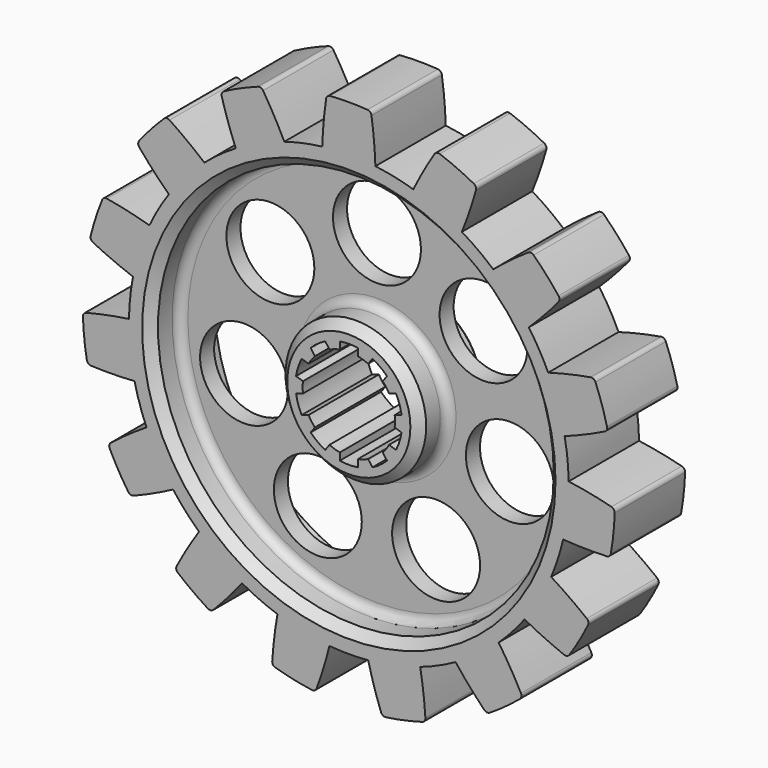
from build123d import *

# Parameters (mm, degrees)
F1_DEPTH  = 20
F2_DEPTH  = 20
F3_R      = 1
F4_COUNT  = 15
F5_R      = 10
F6_DEPTH  = 25
F7_R      = 45
F7_R_2    = 10
F7_R_3    = 16
F8_DEPTH  = 8
F9_R      = 2
F10_SIZE  = 2
F11_R     = 45
F11_R_2   = 16
F12_DEPTH = 8
F13_SIZE  = 2
F14_R     = 2


with BuildPart() as f1:
    # F0 (on Front) → F1 (new body)
    with BuildSketch(Plane.XZ):
        with BuildLine():
            ThreePointArc((-6.0454455831, 49.6331803102), (0, 50), (6.0454455831, 49.6331803102))
            ThreePointArc((6.0454455831, 49.6331803102), (5.6999328162, 54.9765582241), (5.0372687356, 60.2899321917))
            ThreePointArc((5.0372687356, 60.2899321917), (0, 60.5), (-5.0372687356, 60.2899321917))
            ThreePointArc((-5.0372687356, 60.2899321917), (-5.6999328162, 54.9765582241), (-6.0454455831, 49.6331803102))
        make_face()
    extrude(amount=F1_DEPTH)

    # F3
    f3_edges = [f1.edges().sort_by_distance(p)[0] for p in [
        (-5.037269, -10, 60.289932),
        (5.037269, -10, 60.289932),
    ]]
    fillet(f3_edges, radius=F3_R)



with BuildPart() as f2:
    # F0 (on Front) → F2 (new body)
    with BuildSketch(Plane.XZ):
        with BuildLine():
            ThreePointArc((-6.0454455831, 49.6331803102), (-33.14911553, -37.4317530925), (50, 0))
            ThreePointArc((50, 0), (37.4317530925, 33.14911553), (6.0454455831, 49.6331803102))
            ThreePointArc((6.0454455831, 49.6331803102), (0, 50), (-6.0454455831, 49.6331803102))
        make_face()
        with BuildLine():
            ThreePointArc((10.4274046286, 1.2325715847), (10.4818354452, 0.6173537882), (10.5, 0))
            ThreePointArc((10.5, 0), (10.4818354452, -0.6173537882), (10.4274046286, -1.2325715847))
            Line((10.4274046286, -1.2325715847), (11.9961998639, -1.742304056))
            ThreePointArc((11.9961998639, -1.742304056), (11.5230272808, -3.7440585238), (10.729230187, -5.6416357729))
            Line((10.729230187, -5.6416357729), (9.1604349517, -5.1319033015))
            ThreePointArc((9.1604349517, -5.1319033015), (8.4946784409, -6.1717451491), (7.7114601519, -7.1262460192))
            Line((7.7114601519, -7.1262460192), (8.6810289287, -8.4607429543))
            ThreePointArc((8.6810289287, -8.4607429543), (7.1216225128, -9.8020724711), (5.3640592517, -10.8706624887))
            Line((5.3640592517, -10.8706624887), (4.3944904749, -9.5361655536))
            ThreePointArc((4.3944904749, -9.5361655536), (3.2446784409, -9.9860934211), (2.05, -10.2979366865))
            Line((2.05, -10.2979366865), (2.05, -11.947465614))
            ThreePointArc((2.05, -11.947465614), (0, -12.1160278946), (-2.05, -11.947465614))
            Line((-2.05, -11.947465614), (-2.05, -10.2979366865))
            ThreePointArc((-2.05, -10.2979366865), (-3.2446784409, -9.9860934211), (-4.3944904749, -9.5361655536))
            Line((-4.3944904749, -9.5361655536), (-5.3640592517, -10.8706624887))
            ThreePointArc((-5.3640592517, -10.8706624887), (-7.1216225128, -9.8020724711), (-8.6810289287, -8.4607429543))
            Line((-8.6810289287, -8.4607429543), (-7.7114601519, -7.1262460192))
            ThreePointArc((-7.7114601519, -7.1262460192), (-8.4946784409, -6.1717451491), (-9.1604349517, -5.1319033015))
            Line((-9.1604349517, -5.1319033015), (-10.729230187, -5.6416357729))
            ThreePointArc((-10.729230187, -5.6416357729), (-11.5230272808, -3.7440585238), (-11.9961998639, -1.742304056))
            Line((-11.9961998639, -1.742304056), (-10.4274046286, -1.2325715847))
            ThreePointArc((-10.4274046286, -1.2325715847), (-10.5, 0), (-10.4274046286, 1.2325715847))
            Line((-10.4274046286, 1.2325715847), (-11.9961998639, 1.742304056))
            ThreePointArc((-11.9961998639, 1.742304056), (-11.5230272808, 3.7440585238), (-10.729230187, 5.6416357729))
            Line((-10.729230187, 5.6416357729), (-9.1604349517, 5.1319033015))
            ThreePointArc((-9.1604349517, 5.1319033015), (-8.4946784409, 6.1717451491), (-7.7114601519, 7.1262460192))
            Line((-7.7114601519, 7.1262460192), (-8.6810289287, 8.4607429543))
            ThreePointArc((-8.6810289287, 8.4607429543), (-7.1216225128, 9.8020724711), (-5.3640592517, 10.8706624887))
            Line((-5.3640592517, 10.8706624887), (-4.3944904749, 9.5361655536))
            ThreePointArc((-4.3944904749, 9.5361655536), (-3.2446784409, 9.9860934211), (-2.05, 10.2979366865))
            Line((-2.05, 10.2979366865), (-2.05, 11.947465614))
            ThreePointArc((-2.05, 11.947465614), (0, 12.1160278946), (2.05, 11.947465614))
            Line((2.05, 11.947465614), (2.05, 10.2979366865))
            ThreePointArc((2.05, 10.2979366865), (3.2446784409, 9.9860934211), (4.3944904749, 9.5361655536))
            Line((4.3944904749, 9.5361655536), (5.3640592517, 10.8706624887))
            ThreePointArc((5.3640592517, 10.8706624887), (7.1216225128, 9.8020724711), (8.6810289287, 8.4607429543))
            Line((8.6810289287, 8.4607429543), (7.7114601519, 7.1262460192))
            ThreePointArc((7.7114601519, 7.1262460192), (8.4946784409, 6.1717451491), (9.1604349517, 5.1319033015))
            Line((9.1604349517, 5.1319033015), (10.729230187, 5.6416357729))
            ThreePointArc((10.729230187, 5.6416357729), (11.5230272808, 3.7440585238), (11.9961998639, 1.742304056))
            Line((11.9961998639, 1.742304056), (10.4274046286, 1.2325715847))
        make_face(mode=Mode.SUBTRACT)
    extrude(amount=F2_DEPTH)


with BuildPart() as f1_1:
    add(f1.part)

    add(f2.part)  # F4 merges F2
    # F4: F1 ×15 about axis
    f4_axis = Axis((0, 0, 0), (0, -1, 0))
    for i in range(1, F4_COUNT):
        add(f1.part.rotate(f4_axis, i * 360 / F4_COUNT))

    # F5 (on face) → F6 (cut)
    with BuildSketch(Plane.XZ.offset(20)):
        with Locations((0, 31)):
            Circle(F5_R)
        with Locations((24.2367759565, 19.3281838576)):
            Circle(F5_R)
        with Locations((30.2227652776, -6.8981489526)):
            Circle(F5_R)
        with Locations((13.4503959126, -27.930034905)):
            Circle(F5_R)
        with Locations((-13.4503959126, -27.930034905)):
            Circle(F5_R)
        with Locations((-30.2227652776, -6.8981489526)):
            Circle(F5_R)
        with Locations((-24.2367759565, 19.3281838576)):
            Circle(F5_R)
    extrude(amount=-F6_DEPTH, mode=Mode.SUBTRACT)

    # F7 (on face) → F8 (cut)
    with BuildSketch(Plane.XZ.offset(20)):
        Circle(F7_R)
        with Locations((-13.4503959126, -27.930034905)):
            Circle(F7_R_2, mode=Mode.SUBTRACT)
        with Locations((-30.2227652776, -6.8981489526)):
            Circle(F7_R_2, mode=Mode.SUBTRACT)
        with Locations((13.4503959126, -27.930034905)):
            Circle(F7_R_2, mode=Mode.SUBTRACT)
        Circle(F7_R_3, mode=Mode.SUBTRACT)
        with Locations((30.2227652776, -6.8981489526)):
            Circle(F7_R_2, mode=Mode.SUBTRACT)
        with Locations((-24.2367759565, 19.3281838576)):
            Circle(F7_R_2, mode=Mode.SUBTRACT)
        with Locations((24.2367759565, 19.3281838576)):
            Circle(F7_R_2, mode=Mode.SUBTRACT)
        with Locations((0, 31)):
            Circle(F7_R_2, mode=Mode.SUBTRACT)
    extrude(amount=-F8_DEPTH, mode=Mode.SUBTRACT)

    # F9
    f9_edges = [f1_1.edges().sort_by_distance(p)[0] for p in [
        (-16, -12, 0),
        (-45, -12, 0),
    ]]
    fillet(f9_edges, radius=F9_R)

    # F10
    f10_edges = [f1_1.edges().sort_by_distance(p)[0] for p in [
        (-16, -20, 0),
        (-45, -20, 0),
    ]]
    chamfer(f10_edges, length=F10_SIZE)

    # F11 (on face) → F12 (cut)
    with BuildSketch(Plane.XZ):
        with Locations((0, -0.7721988368)):
            Circle(F11_R)
        Circle(F11_R_2, mode=Mode.SUBTRACT)
    extrude(amount=F12_DEPTH, mode=Mode.SUBTRACT)

    # F13
    f13_edges = [f1_1.edges().sort_by_distance(p)[0] for p in [
        (-45, 0, -0.772199),
        (-16, 0, 0),
    ]]
    chamfer(f13_edges, length=F13_SIZE)

    # F14
    f14_edges = [f1_1.edges().sort_by_distance(p)[0] for p in [
        (-45, -8, -0.772199),
        (-16, -8, 0),
    ]]
    fillet(f14_edges, radius=F14_R)


solid = f1_1.part
